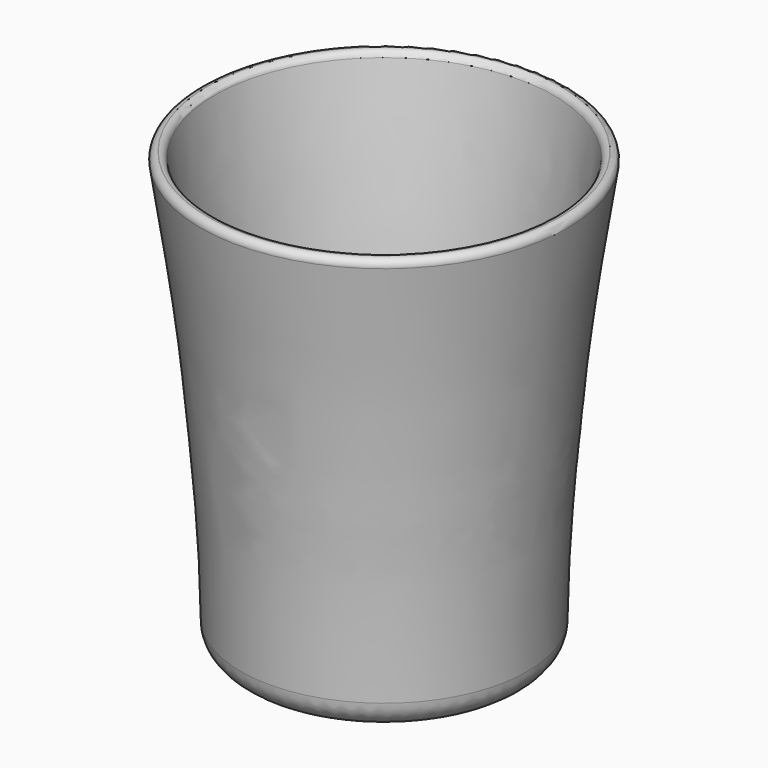
from build123d import *

# Parameters (mm, degrees)
F2_R = 6
F3_T = -3


# Not quite as in the source:
# - a fillet or chamfer that OpenCascade refuses, or shapes differently, is made with other operations: its cross-section is extruded or revolved along the edge and cut away or added


with BuildPart() as f1:
    # F0 (on Front) → F1 (revolve)
    with BuildSketch(Plane.XZ):
        with BuildLine():
            Line((0, 0), (31, 0))
            add(Edge.make_bspline(
                [(31, 0), (31.0335964643, 20.6619363198), (33.7904500865, 46.6403635335), (34.9055384881, 63.2827135687), (40, 95)],
                knots=[0, 0, 0, 0, 0.4771223932, 1, 1, 1, 1], degree=3))
            Line((40, 95), (0, 95))
            Line((0, 95), (0, 0))
        make_face()
    revolve(axis=Axis((0, 0, 47.5), (0, 0, 1)))

    # F2
    f2_edges = [f1.edges().sort_by_distance(p)[0] for p in [
        (-31, 0, 0),
    ]]
    fillet(f2_edges, radius=F2_R)

    # F3
    f3_openings = [f1.faces().sort_by_distance(p)[0] for p in [
        (0, 0, 95),
    ]]
    offset(amount=F3_T, openings=f3_openings)

    # F4: fillet of radius 1.5 on 2 edges, made by hand

    # F4_s1 → F4_t2 (revolve, cut)
    with BuildSketch(Plane.XZ):
        with BuildLine():
            ThreePointArc((39.7221731804, 93.2625963352), (39.3818860804, 94.4734661898), (38.2398082045, 95.0004))
            Line((38.2398082045, 95.0004), (38.2398082045, 95.1505138364))
            ThreePointArc((38.2398082045, 95.1505138364), (39.1199041022, 95.1501138364), (40, 95.1501138364))
            Line((40, 95.1501138364), (40.1482141159, 94.976193704))
            ThreePointArc((40.1482141159, 94.976193704), (40.0089095076, 94.10762509), (39.870409678, 93.2389298051))
            Line((39.870409678, 93.2389298051), (39.7221731804, 93.2625963352))
        make_face()
    revolve(axis=Axis((0, 0, 95), (0, 0, 1)), mode=Mode.SUBTRACT)

    # F4_s3 → F4_t4 (revolve, cut)
    with BuildSketch(Plane.XZ):
        with BuildLine():
            ThreePointArc((38.2417604202, 95.0004), (37.2672082694, 94.6412113654), (36.7588666118, 93.7354756815))
            Line((36.7588666118, 93.7354756815), (36.6105772309, 93.7591506361))
            ThreePointArc((36.6105772309, 93.7591506361), (36.7120450386, 94.3914504759), (36.8133361374, 95.0237774112))
            Line((36.8133361374, 95.0237774112), (36.9616091244, 95.1501673864))
            ThreePointArc((36.9616091244, 95.1501673864), (37.6016847723, 95.1501673864), (38.2417604202, 95.1505673864))
            Line((38.2417604202, 95.1505673864), (38.2417604202, 95.0004))
        make_face()
    revolve(axis=Axis((-6e-10, 1e-10, 95), (0, 0, -1)), mode=Mode.SUBTRACT)


solid = f1.part
